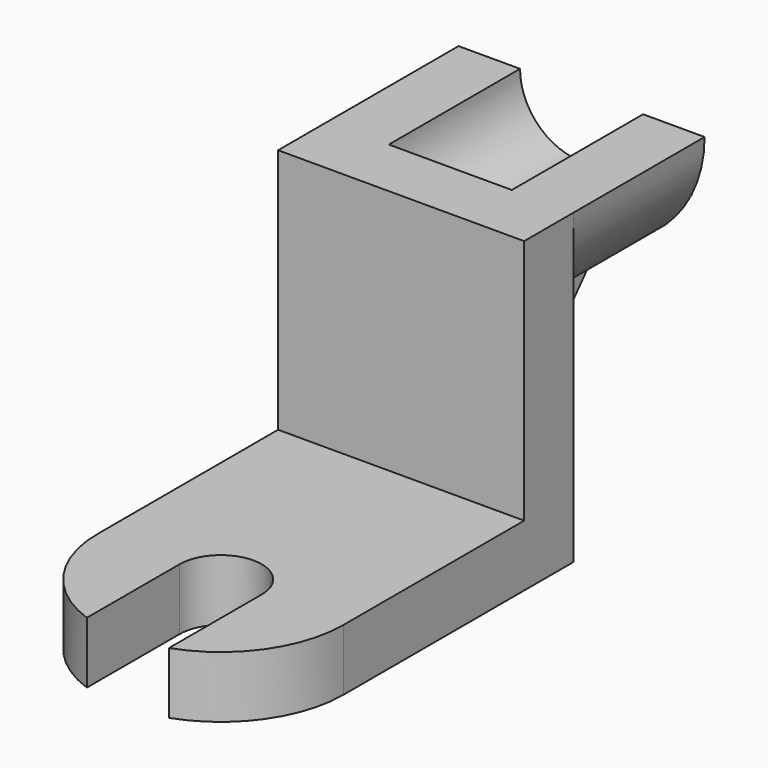
from build123d import *

# Parameters (mm, degrees)
F0_W      = 60
F0_H      = 15
F1_DEPTH  = 75
F2_DEPTH  = 15
F4_DEPTH  = 25
F6_DEPTH  = 40
F8_DEPTH  = 40
F10_DEPTH = 25


with BuildPart() as f1:
    # F0 (on Top) → F1 (new body)
    with BuildSketch(Plane.XY):
        with Locations((17.5909090042, 32.8136347234)):
            Rectangle(F0_W, F0_H)
    extrude(amount=F1_DEPTH)

    # F0 (on Top) → F2 (join)
    with BuildSketch(Plane.XY):
        with Locations((17.5909090042, 32.8136347234)):
            Rectangle(F0_W, F0_H)
        with BuildLine():
            Line((47.5909090042, 25.3136347234), (-12.4090909958, 25.3136347234))
            Line((-12.4090909958, 25.3136347234), (-12.4090909958, -29.6863652766))
            ThreePointArc((-12.4090909958, -29.6863652766), (17.5909090042, 0.3136347234), (47.5909090042, -29.6863652766))
            Line((47.5909090042, -29.6863652766), (47.5909090042, 25.3136347234))
        make_face()
        with BuildLine():
            ThreePointArc((47.5909090042, -29.6863652766), (17.5909090042, 0.3136347234), (-12.4090909958, -29.6863652766))
            Line((-12.4090909958, -29.6863652766), (47.5909090042, -29.6863652766))
        make_face()
        with BuildLine():
            Line((47.5909090042, -29.6863652766), (-12.4090909958, -29.6863652766))
            ThreePointArc((-12.4090909958, -29.6863652766), (17.5909090042, -59.6863652766), (47.5909090042, -29.6863652766))
        make_face()
    extrude(amount=F2_DEPTH)

    # F3 (on face) → F4 (cut)
    with BuildSketch(Plane.XY.offset(15)):
        with BuildLine():
            ThreePointArc((7.5909090042, -57.970636524), (17.5909090042, -59.6863652766), (27.5909090042, -57.970636524))
            Line((27.5909090042, -57.970636524), (27.5909090042, -29.6863652766))
            ThreePointArc((27.5909090042, -29.6863652766), (17.5909090042, -39.6863652766), (7.5909090042, -29.6863652766))
            Line((7.5909090042, -29.6863652766), (7.5909090042, -57.970636524))
        make_face()
        with BuildLine():
            ThreePointArc((7.5909090042, -29.6863652766), (17.5909090042, -39.6863652766), (27.5909090042, -29.6863652766))
            Line((27.5909090042, -29.6863652766), (17.5909090042, -29.6863652766))
            Line((17.5909090042, -29.6863652766), (7.5909090042, -29.6863652766))
        make_face()
        with BuildLine():
            Line((17.5909090042, -29.6863652766), (27.5909090042, -29.6863652766))
            ThreePointArc((27.5909090042, -29.6863652766), (17.5909090042, -19.6863652766), (7.5909090042, -29.6863652766))
            Line((7.5909090042, -29.6863652766), (17.5909090042, -29.6863652766))
        make_face()
    extrude(amount=-F4_DEPTH, mode=Mode.SUBTRACT)

    # F5 (on face) → F6 (join)
    with BuildSketch(Plane(origin=(0, 40.3136347234, 0), x_dir=(-1, 0, 0), z_dir=(0, 1, 0))):
        with BuildLine():
            Line((-42.2313958406, 75), (-47.5909090042, 75))
            ThreePointArc((-47.5909090042, 75), (-17.5909090042, 45), (12.4090909958, 75))
            Line((12.4090909958, 75), (-2.5909090042, 75))
            ThreePointArc((-2.5909090042, 75), (-17.5909090042, 60), (-32.5909090042, 75))
            Line((-32.5909090042, 75), (-42.2313958406, 75))
        make_face()
    extrude(amount=F6_DEPTH)

    # F7 (on face) → F8 (join)
    with BuildSketch(Plane(origin=(0, 40.3136347234, 0), x_dir=(-1, 0, 0), z_dir=(0, 1, 0))):
        with BuildLine():
            Line((-22.5909090042, 45.4196010845), (-22.5909090042, 0))
            Line((-22.5909090042, 0), (-12.5909090042, 0))
            Line((-12.5909090042, 0), (-12.5909090042, 45.4196010845))
            ThreePointArc((-12.5909090042, 45.4196010845), (-17.5909090042, 45), (-22.5909090042, 45.4196010845))
        make_face()
    extrude(amount=F8_DEPTH)

    # F9 (on face) → F10 (cut)
    with BuildSketch(Plane(origin=(12.5909090042, 0, 0), x_dir=(0, -1, 0), z_dir=(-1, 0, 0))):
        Polygon((-40.3136347234, 0), (-80.3136347234, 45.4196010845), (-80.3136347234, 0), align=None)
    extrude(amount=-F10_DEPTH, mode=Mode.SUBTRACT)


solid = f1.part
